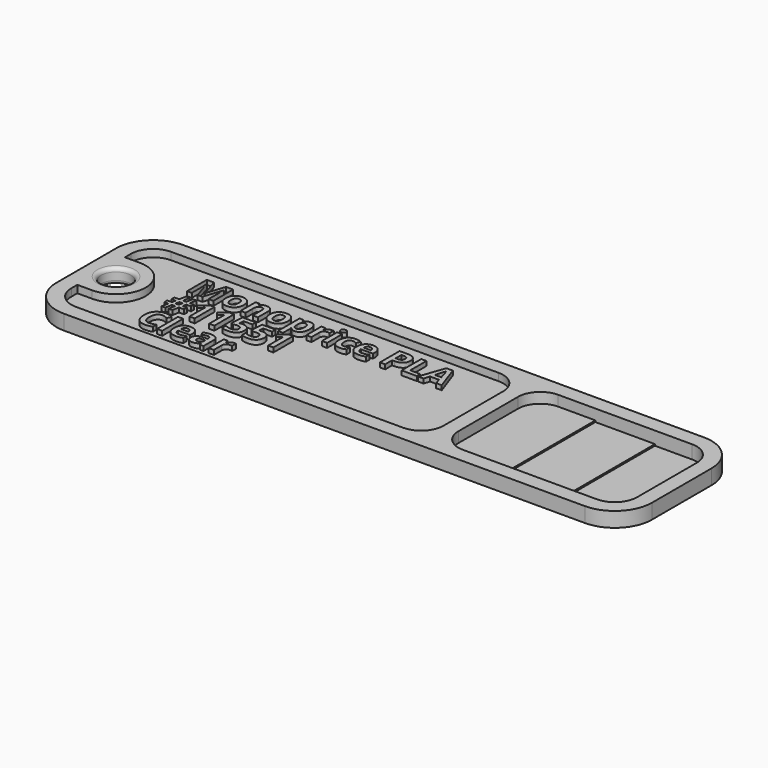
from build123d import *

# Parameters (mm, degrees)
F1_DEPTH      = 2
F3_DEPTH      = 1
F4_R          = 2
F5_DEPTH      = 2.001
F6_R          = 0.5
F7_DEPTH      = 0.4
F9_DEPTH      = 0.2
F11_DEPTH     = 0.2
F12_TEXT_SIZE = 4.6296296296
F13_DEPTH     = 0.6


# Not quite as in the source:
# - Text() gives the source's letters only with a copy of the font that has no kerning and outlines rounded to 1/6400 em; it was checked with that copy


with BuildPart() as f1:
    # F0 (on Top) → F1 (new body)
    with BuildSketch(Plane.XY):
        with BuildLine():
            ThreePointArc((40, 5), (38.5355339059, 8.5355339059), (35, 10))
            Line((35, 10), (-35, 10))
            ThreePointArc((-35, 10), (-38.5355339059, 8.5355339059), (-40, 5))
            Line((-40, 5), (-40, -5))
            ThreePointArc((-40, -5), (-38.5355339059, -8.5355339059), (-35, -10))
            Line((-35, -10), (35, -10))
            ThreePointArc((35, -10), (38.5355339059, -8.5355339059), (40, -5))
            Line((40, -5), (40, 5))
        make_face()
    extrude(amount=F1_DEPTH)

    # F2 (on face) → F3 (cut)
    with BuildSketch(Plane.XY.offset(2)):
        with BuildLine():
            ThreePointArc((35, -8), (37.1213203436, -7.1213203436), (38, -5))
            Line((38, -5), (38, 5))
            ThreePointArc((38, 5), (37.1213203436, 7.1213203436), (35, 8))
            Line((35, 8), (17, 8))
            ThreePointArc((17, 8), (14.8786796564, 7.1213203436), (14, 5))
            Line((14, 5), (14, -5))
            ThreePointArc((14, -5), (14.8786796564, -7.1213203436), (17, -8))
            Line((17, -8), (35, -8))
        make_face()
        with BuildLine():
            ThreePointArc((-38, -5), (-37.1213203436, -7.1213203436), (-35, -8))
            Line((-35, -8), (9, -8))
            ThreePointArc((9, -8), (11.1213203436, -7.1213203436), (12, -5))
            Line((12, -5), (12, 5))
            ThreePointArc((12, 5), (11.1213203436, 7.1213203436), (9, 8))
            Line((9, 8), (-35, 8))
            ThreePointArc((-35, 8), (-37.1213203436, 7.1213203436), (-38, 5))
            Line((-38, 5), (-38, 4))
            Line((-38, 4), (-36, 4))
            ThreePointArc((-36, 4), (-32, 0), (-36, -4))
            Line((-36, -4), (-38, -4))
            Line((-38, -4), (-38, -5))
        make_face()
    extrude(amount=-F3_DEPTH, mode=Mode.SUBTRACT)

    # F4 (on face) → F5 (cut, through all)
    with BuildSketch(Plane.XY.offset(2)):
        with Locations((-36, 0)):
            Circle(F4_R)
    extrude(amount=-F5_DEPTH, mode=Mode.SUBTRACT)

    # F6
    f6_edges = [f1.edges().sort_by_distance(p)[0] for p in [
        (-38, 0, 2),
        (-38, 0, 0),
    ]]
    fillet(f6_edges, radius=F6_R)

    # F7 (cut): a face of the model
    f7_faces = [f1.faces().sort_by_distance(p)[0] for p in [
        (26, 0, 1),
    ]]
    extrude(f7_faces, amount=-F7_DEPTH, mode=Mode.SUBTRACT)

    # F8 (on face) → F9 (cut)
    with BuildSketch(Plane.XY.offset(0.6)):
        with BuildLine():
            Line((22, -8), (35, -8))
            ThreePointArc((35, -8), (37.1213203436, -7.1213203436), (38, -5))
            Line((38, -5), (38, 5))
            ThreePointArc((38, 5), (37.1213203436, 7.1213203436), (35, 8))
            Line((35, 8), (22, 8))
            Line((22, 8), (22, -8))
        make_face()
    extrude(amount=-F9_DEPTH, mode=Mode.SUBTRACT)

    # F10 (on face) → F11 (cut)
    with BuildSketch(Plane.XY.offset(0.4)):
        with BuildLine():
            ThreePointArc((38, 5), (37.1213203436, 7.1213203436), (35, 8))
            Line((35, 8), (30, 8))
            Line((30, 8), (30, -8))
            Line((30, -8), (35, -8))
            ThreePointArc((35, -8), (37.1213203436, -7.1213203436), (38, -5))
            Line((38, -5), (38, 5))
        make_face()
    extrude(amount=-F11_DEPTH, mode=Mode.SUBTRACT)

    # F12 (on face) → F13 (join)
    with BuildSketch(Plane.XY.offset(1)):
        with Locations((-29, 2.6666666667)):
            Text('Monoprice PLA', F12_TEXT_SIZE, font='Open Sans', font_style=FontStyle.BOLD, text_align=(TextAlign.LEFT, TextAlign.BOTTOM))
        with Locations((-29, -1.6666666667)):
            Text('#11551', F12_TEXT_SIZE, font='Open Sans', font_style=FontStyle.BOLD, text_align=(TextAlign.LEFT, TextAlign.BOTTOM))
        with Locations((-29, -6)):
            Text('Clear', F12_TEXT_SIZE, font='Open Sans', font_style=FontStyle.BOLD, text_align=(TextAlign.LEFT, TextAlign.BOTTOM))
    extrude(amount=F13_DEPTH)


solid = f1.part
